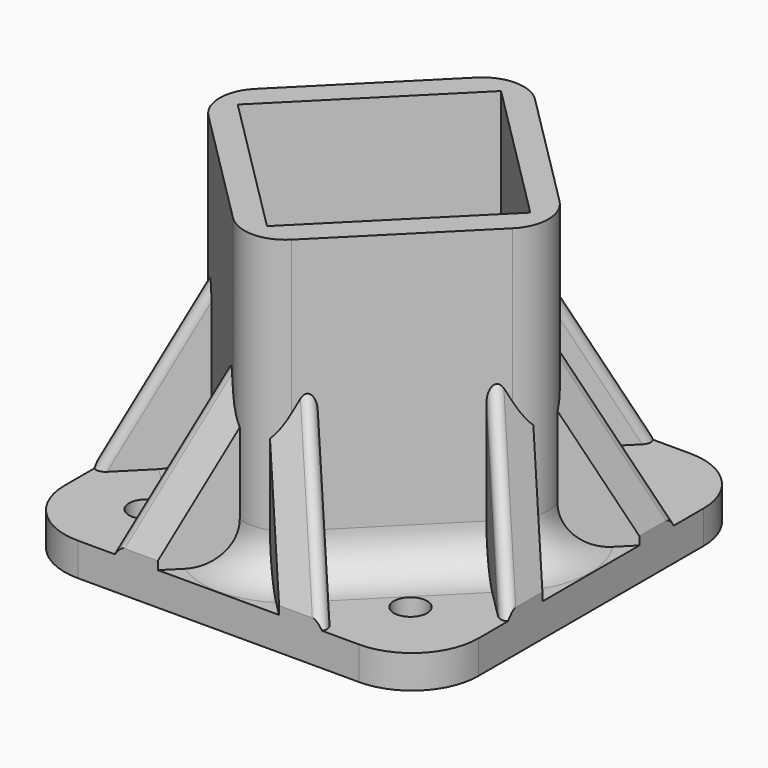
from build123d import *

# Parameters (mm, degrees)
F0_R         = 2
F1_DEPTH     = 4
F0_R_2       = 5
F2_DEPTH     = 40
F3_R         = 8
F4_DEPTH     = 25
F5_T4_DEPTH  = 110.0885065959
F5_T10_DEPTH = 110.0885065959
F5_T16_DEPTH = 110.0885065959
F5_T22_DEPTH = 110.0885065959
F5_T28_DEPTH = 110.0885065959
F5_T34_DEPTH = 110.0885065959
F5_T40_DEPTH = 110.0885065959
F5_T46_DEPTH = 110.0885065959
F5_T52_DEPTH = 110.0885065959
F5_T58_DEPTH = 110.0885065959
F5_T64_DEPTH = 110.0885065959
F5_T70_DEPTH = 110.0885065959
F6_T4_DEPTH  = 110.0885065959
F6_T10_DEPTH = 110.0885065959
F6_T16_DEPTH = 110.0885065959
F6_T22_DEPTH = 110.0885065959
F6_T28_DEPTH = 110.0885065959
F6_T34_DEPTH = 110.0885065959
F6_T40_DEPTH = 110.0885065959
F6_T46_DEPTH = 110.0885065959
F6_T52_DEPTH = 110.0885065959
F6_T58_DEPTH = 110.0885065959
F6_T64_DEPTH = 110.0885065959
F6_T70_DEPTH = 110.0885065959
F7_T4_DEPTH  = 33.9588716378
F7_T10_DEPTH = 33.9588716378
F7_T16_DEPTH = 33.9588716378
F7_T22_DEPTH = 33.9588716378
F7_T28_DEPTH = 33.9588716378
F7_T34_DEPTH = 33.9588716378
F7_T40_DEPTH = 33.9588716378
F7_T46_DEPTH = 33.9588716378
F8_R         = 5
F9_R         = 5


# Not quite as in the source:
# - a fillet or chamfer that OpenCascade refuses, or shapes differently, is made with other operations: its cross-section is extruded or revolved along the edge and cut away or added


with BuildPart() as f1:
    # F0 (on Top) → F1 (new body)
    with BuildSketch(Plane.XY):
        Polygon((16.6170093579, 5.3033008589), (25, 13.686291501), (25, 25), (13.686291501, 25), (5.3033008589, 16.6170093579), align=None)
        with Locations((16, 16)):
            Circle(F0_R, mode=Mode.SUBTRACT)
        Polygon((19.7989898732, -2.1213203436), (25, -7.3223304703), (25, 7.3223304703), (19.7989898732, 2.1213203436), (21.9203102168, 0), align=None)
        Polygon((13.686291501, -25), (25, -25), (25, -13.686291501), (16.6170093579, -5.3033008589), (5.3033008589, -16.6170093579), align=None)
        with Locations((16, -16)):
            Circle(F0_R, mode=Mode.SUBTRACT)
        Polygon((-7.3223304703, -25), (7.3223304703, -25), (2.1213203436, -19.7989898732), (0, -21.9203102168), (-2.1213203436, -19.7989898732), align=None)
        Polygon((-25, -25), (-13.686291501, -25), (-5.3033008589, -16.6170093579), (-16.6170093579, -5.3033008589), (-25, -13.686291501), align=None)
        with Locations((-16, -16)):
            Circle(F0_R, mode=Mode.SUBTRACT)
        Polygon((-25, 7.3223304703), (-25, -7.3223304703), (-19.7989898732, -2.1213203436), (-21.9203102168, 0), (-19.7989898732, 2.1213203436), align=None)
        Polygon((-25, 25), (-25, 13.686291501), (-16.6170093579, 5.3033008589), (-5.3033008589, 16.6170093579), (-13.686291501, 25), align=None)
        with Locations((-16, 16)):
            Circle(F0_R, mode=Mode.SUBTRACT)
        Polygon((-2.1213203436, 19.7989898732), (-7.3223304703, 25), (-13.686291501, 25), (-5.3033008589, 16.6170093579), align=None)
        Polygon((2.1213203436, 19.7989898732), (7.3223304703, 25), (-7.3223304703, 25), (-2.1213203436, 19.7989898732), (0, 21.9203102168), align=None)
        Polygon((5.3033008589, 16.6170093579), (13.686291501, 25), (7.3223304703, 25), (2.1213203436, 19.7989898732), align=None)
        Polygon((19.7989898732, 2.1213203436), (25, 7.3223304703), (25, 13.686291501), (16.6170093579, 5.3033008589), align=None)
        Polygon((16.6170093579, -5.3033008589), (25, -13.686291501), (25, -7.3223304703), (19.7989898732, -2.1213203436), align=None)
        Polygon((7.3223304703, -25), (13.686291501, -25), (5.3033008589, -16.6170093579), (2.1213203436, -19.7989898732), align=None)
        Polygon((-13.686291501, -25), (-7.3223304703, -25), (-2.1213203436, -19.7989898732), (-5.3033008589, -16.6170093579), align=None)
        Polygon((-25, -7.3223304703), (-25, -13.686291501), (-16.6170093579, -5.3033008589), (-19.7989898732, -2.1213203436), align=None)
        Polygon((-25, 13.686291501), (-25, 7.3223304703), (-19.7989898732, 2.1213203436), (-16.6170093579, 5.3033008589), align=None)
    extrude(amount=F1_DEPTH)



with BuildPart() as f1b:
    # F0 (on Top) → F1, piece 2 (new body)
    with BuildSketch(Plane.XY):
        Polygon((0, -17.6776695297), (17.6776695297, 0), (0, 17.6776695297), (-17.6776695297, 0), align=None)
        Circle(F0_R_2, mode=Mode.SUBTRACT)
    extrude(amount=F1_DEPTH)


with BuildPart() as f1_1:
    add(f1.part)

    add(f1b.part)  # F2 merges F1b
    # F0 (on Top) → F2 (join)
    with BuildSketch(Plane.XY):
        Polygon((2.1213203436, -19.7989898732), (5.3033008589, -16.6170093579), (16.6170093579, -5.3033008589), (19.7989898732, -2.1213203436), (21.9203102168, 0), (19.7989898732, 2.1213203436), (16.6170093579, 5.3033008589), (5.3033008589, 16.6170093579), (2.1213203436, 19.7989898732), (0, 21.9203102168), (-2.1213203436, 19.7989898732), (-5.3033008589, 16.6170093579), (-16.6170093579, 5.3033008589), (-19.7989898732, 2.1213203436), (-21.9203102168, 0), (-19.7989898732, -2.1213203436), (-16.6170093579, -5.3033008589), (-5.3033008589, -16.6170093579), (-2.1213203436, -19.7989898732), (0, -21.9203102168), align=None)
        Polygon((0, 17.6776695297), (17.6776695297, 0), (0, -17.6776695297), (-17.6776695297, 0), align=None, mode=Mode.SUBTRACT)
    extrude(amount=F2_DEPTH)

    # F3
    f3_edges = [f1_1.edges().sort_by_distance(p)[0] for p in [
        (-25, 25, 2),
        (-25, -25, 2),
        (25, -25, 2),
        (25, 25, 2),
    ]]
    fillet(f3_edges, radius=F3_R)

    # F0 (on Top) → F4 (join)
    with BuildSketch(Plane.XY):
        Polygon((16.6170093579, -5.3033008589), (25, -13.686291501), (25, -7.3223304703), (19.7989898732, -2.1213203436), align=None)
        Polygon((7.3223304703, -25), (13.686291501, -25), (5.3033008589, -16.6170093579), (2.1213203436, -19.7989898732), align=None)
        Polygon((5.3033008589, 16.6170093579), (13.686291501, 25), (7.3223304703, 25), (2.1213203436, 19.7989898732), align=None)
        Polygon((19.7989898732, 2.1213203436), (25, 7.3223304703), (25, 13.686291501), (16.6170093579, 5.3033008589), align=None)
        Polygon((-13.686291501, -25), (-7.3223304703, -25), (-2.1213203436, -19.7989898732), (-5.3033008589, -16.6170093579), align=None)
        Polygon((-25, -7.3223304703), (-25, -13.686291501), (-16.6170093579, -5.3033008589), (-19.7989898732, -2.1213203436), align=None)
        Polygon((-25, 13.686291501), (-25, 7.3223304703), (-19.7989898732, 2.1213203436), (-16.6170093579, 5.3033008589), align=None)
        Polygon((-2.1213203436, 19.7989898732), (-7.3223304703, 25), (-13.686291501, 25), (-5.3033008589, 16.6170093579), align=None)
    extrude(amount=F4_DEPTH)

    # F5: chamfer of 20 x 8 on 4 edges, made by hand


with BuildPart() as f5_tool2:
    # F5_s3 → F5_t4 (new body)
    with BuildSketch(Plane.YZ.offset(-65.5485642836)):
        Polygon((-17, 25), (-25, 5), (-25, 25), align=None)
    extrude(amount=F5_T4_DEPTH)

    split(bisect_by=Plane(origin=(-10.9601551084, -10.9601551084, 0), x_dir=(0, 0, 1), z_dir=(-0.7071067812, -0.7071067812, 0)), keep=Keep.TOP)

    split(bisect_by=Plane(origin=(10.9601551084, -10.9601551084, 0), x_dir=(0, 0, 1), z_dir=(-0.7071067812, 0.7071067812, 0)), keep=Keep.TOP)


with BuildPart() as f1_2:
    add(f1_1.part)

    # F5_t1: cut F5_tool2
    add(f5_tool2.part, mode=Mode.SUBTRACT)


with BuildPart() as f5_tool8:
    # F5_s9 → F5_t10 (new body)
    with BuildSketch(Plane.YZ.offset(-65.5485642836)):
        Polygon((-17, 25), (-25, 5), (-25, 25), align=None)
    extrude(amount=F5_T10_DEPTH)

    split(bisect_by=Plane(origin=(-10.9601551084, -10.9601551084, 0), x_dir=(0, 0, 1), z_dir=(-0.7071067812, -0.7071067812, 0)), keep=Keep.TOP)

    split(bisect_by=Plane(origin=(10.9601551084, -10.9601551084, 0), x_dir=(0, 0, 1), z_dir=(0.7071067812, -0.7071067812, 0)), keep=Keep.TOP)


with BuildPart() as f1_3:
    add(f1_2.part)

    # F5_t7: cut F5_tool8
    add(f5_tool8.part, mode=Mode.SUBTRACT)


with BuildPart() as f5_tool14:
    # F5_s15 → F5_t16 (new body)
    with BuildSketch(Plane.YZ.offset(-65.5485642836)):
        Polygon((-17, 25), (-25, 5), (-25, 25), align=None)
    extrude(amount=F5_T16_DEPTH)

    split(bisect_by=Plane(origin=(-10.9601551084, -10.9601551084, 0), x_dir=(0, 0, 1), z_dir=(0.7071067812, 0.7071067812, 0)), keep=Keep.TOP)

    split(bisect_by=Plane(origin=(10.9601551084, -10.9601551084, 0), x_dir=(0, 0, 1), z_dir=(0.7071067812, -0.7071067812, 0)), keep=Keep.TOP)


with BuildPart() as f1_4:
    add(f1_3.part)

    # F5_t13: cut F5_tool14
    add(f5_tool14.part, mode=Mode.SUBTRACT)


with BuildPart() as f5_tool20:
    # F5_s21 → F5_t22 (new body)
    with BuildSketch(Plane.YZ.offset(-44.5399423123)):
        Polygon((-17, 25), (-25, 5), (-25, 25), align=None)
    extrude(amount=F5_T22_DEPTH)

    split(bisect_by=Plane(origin=(-10.9601551084, -10.9601551084, 0), x_dir=(0, 0, 1), z_dir=(-0.7071067812, -0.7071067812, 0)), keep=Keep.TOP)

    split(bisect_by=Plane(origin=(10.9601551084, -10.9601551084, 0), x_dir=(0, 0, 1), z_dir=(-0.7071067812, 0.7071067812, 0)), keep=Keep.TOP)


with BuildPart() as f1_5:
    add(f1_4.part)

    # F5_t19: cut F5_tool20
    add(f5_tool20.part, mode=Mode.SUBTRACT)


with BuildPart() as f5_tool26:
    # F5_s27 → F5_t28 (new body)
    with BuildSketch(Plane.YZ.offset(-44.5399423123)):
        Polygon((-17, 25), (-25, 5), (-25, 25), align=None)
    extrude(amount=F5_T28_DEPTH)

    split(bisect_by=Plane(origin=(-10.9601551084, -10.9601551084, 0), x_dir=(0, 0, 1), z_dir=(-0.7071067812, -0.7071067812, 0)), keep=Keep.TOP)

    split(bisect_by=Plane(origin=(10.9601551084, -10.9601551084, 0), x_dir=(0, 0, 1), z_dir=(0.7071067812, -0.7071067812, 0)), keep=Keep.TOP)


with BuildPart() as f1_6:
    add(f1_5.part)

    # F5_t25: cut F5_tool26
    add(f5_tool26.part, mode=Mode.SUBTRACT)


with BuildPart() as f5_tool32:
    # F5_s33 → F5_t34 (new body)
    with BuildSketch(Plane.YZ.offset(-44.5399423123)):
        Polygon((-17, 25), (-25, 5), (-25, 25), align=None)
    extrude(amount=F5_T34_DEPTH)

    split(bisect_by=Plane(origin=(-10.9601551084, -10.9601551084, 0), x_dir=(0, 0, 1), z_dir=(0.7071067812, 0.7071067812, 0)), keep=Keep.TOP)

    split(bisect_by=Plane(origin=(10.9601551084, -10.9601551084, 0), x_dir=(0, 0, 1), z_dir=(0.7071067812, -0.7071067812, 0)), keep=Keep.TOP)


with BuildPart() as f1_7:
    add(f1_6.part)

    # F5_t31: cut F5_tool32
    add(f5_tool32.part, mode=Mode.SUBTRACT)


with BuildPart() as f5_tool38:
    # F5_s39 → F5_t40 (new body)
    with BuildSketch(Plane.XZ.offset(-65.5485642836)):
        Polygon((-17, 25), (-25, 5), (-25, 25), align=None)
    extrude(amount=F5_T40_DEPTH)

    split(bisect_by=Plane(origin=(-10.9601551084, 10.9601551084, 0), x_dir=(0, 0, 1), z_dir=(-0.7071067812, 0.7071067812, 0)), keep=Keep.TOP)

    split(bisect_by=Plane(origin=(-10.9601551084, -10.9601551084, 0), x_dir=(0, 0, 1), z_dir=(0.7071067812, 0.7071067812, 0)), keep=Keep.TOP)


with BuildPart() as f1_8:
    add(f1_7.part)

    # F5_t37: cut F5_tool38
    add(f5_tool38.part, mode=Mode.SUBTRACT)


with BuildPart() as f5_tool44:
    # F5_s45 → F5_t46 (new body)
    with BuildSketch(Plane.XZ.offset(-65.5485642836)):
        Polygon((-17, 25), (-25, 5), (-25, 25), align=None)
    extrude(amount=F5_T46_DEPTH)

    split(bisect_by=Plane(origin=(-10.9601551084, 10.9601551084, 0), x_dir=(0, 0, 1), z_dir=(-0.7071067812, 0.7071067812, 0)), keep=Keep.TOP)

    split(bisect_by=Plane(origin=(-10.9601551084, -10.9601551084, 0), x_dir=(0, 0, 1), z_dir=(-0.7071067812, -0.7071067812, 0)), keep=Keep.TOP)


with BuildPart() as f1_9:
    add(f1_8.part)

    # F5_t43: cut F5_tool44
    add(f5_tool44.part, mode=Mode.SUBTRACT)


with BuildPart() as f5_tool50:
    # F5_s51 → F5_t52 (new body)
    with BuildSketch(Plane.XZ.offset(-65.5485642836)):
        Polygon((-17, 25), (-25, 5), (-25, 25), align=None)
    extrude(amount=F5_T52_DEPTH)

    split(bisect_by=Plane(origin=(-10.9601551084, 10.9601551084, 0), x_dir=(0, 0, 1), z_dir=(0.7071067812, -0.7071067812, 0)), keep=Keep.TOP)

    split(bisect_by=Plane(origin=(-10.9601551084, -10.9601551084, 0), x_dir=(0, 0, 1), z_dir=(-0.7071067812, -0.7071067812, 0)), keep=Keep.TOP)


with BuildPart() as f1_10:
    add(f1_9.part)

    # F5_t49: cut F5_tool50
    add(f5_tool50.part, mode=Mode.SUBTRACT)


with BuildPart() as f5_tool56:
    # F5_s57 → F5_t58 (new body)
    with BuildSketch(Plane.XZ.offset(-44.5399423123)):
        Polygon((-17, 25), (-25, 5), (-25, 25), align=None)
    extrude(amount=F5_T58_DEPTH)

    split(bisect_by=Plane(origin=(-10.9601551084, 10.9601551084, 0), x_dir=(0, 0, 1), z_dir=(-0.7071067812, 0.7071067812, 0)), keep=Keep.TOP)

    split(bisect_by=Plane(origin=(-10.9601551084, -10.9601551084, 0), x_dir=(0, 0, 1), z_dir=(0.7071067812, 0.7071067812, 0)), keep=Keep.TOP)


with BuildPart() as f1_11:
    add(f1_10.part)

    # F5_t55: cut F5_tool56
    add(f5_tool56.part, mode=Mode.SUBTRACT)


with BuildPart() as f5_tool62:
    # F5_s63 → F5_t64 (new body)
    with BuildSketch(Plane.XZ.offset(-44.5399423123)):
        Polygon((-17, 25), (-25, 5), (-25, 25), align=None)
    extrude(amount=F5_T64_DEPTH)

    split(bisect_by=Plane(origin=(-10.9601551084, 10.9601551084, 0), x_dir=(0, 0, 1), z_dir=(-0.7071067812, 0.7071067812, 0)), keep=Keep.TOP)

    split(bisect_by=Plane(origin=(-10.9601551084, -10.9601551084, 0), x_dir=(0, 0, 1), z_dir=(-0.7071067812, -0.7071067812, 0)), keep=Keep.TOP)


with BuildPart() as f1_12:
    add(f1_11.part)

    # F5_t61: cut F5_tool62
    add(f5_tool62.part, mode=Mode.SUBTRACT)


with BuildPart() as f5_tool68:
    # F5_s69 → F5_t70 (new body)
    with BuildSketch(Plane.XZ.offset(-44.5399423123)):
        Polygon((-17, 25), (-25, 5), (-25, 25), align=None)
    extrude(amount=F5_T70_DEPTH)

    split(bisect_by=Plane(origin=(-10.9601551084, 10.9601551084, 0), x_dir=(0, 0, 1), z_dir=(0.7071067812, -0.7071067812, 0)), keep=Keep.TOP)

    split(bisect_by=Plane(origin=(-10.9601551084, -10.9601551084, 0), x_dir=(0, 0, 1), z_dir=(-0.7071067812, -0.7071067812, 0)), keep=Keep.TOP)


with BuildPart() as f1_13:
    add(f1_12.part)

    # F5_t67: cut F5_tool68
    add(f5_tool68.part, mode=Mode.SUBTRACT)

    # F6: chamfer of 8 x 20 on 4 edges, made by hand


with BuildPart() as f6_tool2:
    # F6_s3 → F6_t4 (new body)
    with BuildSketch(Plane.XZ.offset(65.5485642836)):
        Polygon((17, 25), (25, 5), (25, 25), align=None)
    extrude(amount=-F6_T4_DEPTH)

    split(bisect_by=Plane(origin=(10.9601551084, -10.9601551084, 0), x_dir=(0, 0, 1), z_dir=(0.7071067812, -0.7071067812, 0)), keep=Keep.TOP)

    split(bisect_by=Plane(origin=(10.9601551084, 10.9601551084, 0), x_dir=(0, 0, 1), z_dir=(-0.7071067812, -0.7071067812, 0)), keep=Keep.TOP)


with BuildPart() as f1_14:
    add(f1_13.part)

    # F6_t1: cut F6_tool2
    add(f6_tool2.part, mode=Mode.SUBTRACT)


with BuildPart() as f6_tool8:
    # F6_s9 → F6_t10 (new body)
    with BuildSketch(Plane.XZ.offset(65.5485642836)):
        Polygon((17, 25), (25, 5), (25, 25), align=None)
    extrude(amount=-F6_T10_DEPTH)

    split(bisect_by=Plane(origin=(10.9601551084, -10.9601551084, 0), x_dir=(0, 0, 1), z_dir=(0.7071067812, -0.7071067812, 0)), keep=Keep.TOP)

    split(bisect_by=Plane(origin=(10.9601551084, 10.9601551084, 0), x_dir=(0, 0, 1), z_dir=(0.7071067812, 0.7071067812, 0)), keep=Keep.TOP)


with BuildPart() as f1_15:
    add(f1_14.part)

    # F6_t7: cut F6_tool8
    add(f6_tool8.part, mode=Mode.SUBTRACT)


with BuildPart() as f6_tool14:
    # F6_s15 → F6_t16 (new body)
    with BuildSketch(Plane.XZ.offset(65.5485642836)):
        Polygon((17, 25), (25, 5), (25, 25), align=None)
    extrude(amount=-F6_T16_DEPTH)

    split(bisect_by=Plane(origin=(10.9601551084, -10.9601551084, 0), x_dir=(0, 0, 1), z_dir=(-0.7071067812, 0.7071067812, 0)), keep=Keep.TOP)

    split(bisect_by=Plane(origin=(10.9601551084, 10.9601551084, 0), x_dir=(0, 0, 1), z_dir=(0.7071067812, 0.7071067812, 0)), keep=Keep.TOP)


with BuildPart() as f1_16:
    add(f1_15.part)

    # F6_t13: cut F6_tool14
    add(f6_tool14.part, mode=Mode.SUBTRACT)


with BuildPart() as f6_tool20:
    # F6_s21 → F6_t22 (new body)
    with BuildSketch(Plane.XZ.offset(44.5399423123)):
        Polygon((17, 25), (25, 5), (25, 25), align=None)
    extrude(amount=-F6_T22_DEPTH)

    split(bisect_by=Plane(origin=(10.9601551084, -10.9601551084, 0), x_dir=(0, 0, 1), z_dir=(0.7071067812, -0.7071067812, 0)), keep=Keep.TOP)

    split(bisect_by=Plane(origin=(10.9601551084, 10.9601551084, 0), x_dir=(0, 0, 1), z_dir=(-0.7071067812, -0.7071067812, 0)), keep=Keep.TOP)


with BuildPart() as f1_17:
    add(f1_16.part)

    # F6_t19: cut F6_tool20
    add(f6_tool20.part, mode=Mode.SUBTRACT)


with BuildPart() as f6_tool26:
    # F6_s27 → F6_t28 (new body)
    with BuildSketch(Plane.XZ.offset(44.5399423123)):
        Polygon((17, 25), (25, 5), (25, 25), align=None)
    extrude(amount=-F6_T28_DEPTH)

    split(bisect_by=Plane(origin=(10.9601551084, -10.9601551084, 0), x_dir=(0, 0, 1), z_dir=(0.7071067812, -0.7071067812, 0)), keep=Keep.TOP)

    split(bisect_by=Plane(origin=(10.9601551084, 10.9601551084, 0), x_dir=(0, 0, 1), z_dir=(0.7071067812, 0.7071067812, 0)), keep=Keep.TOP)


with BuildPart() as f1_18:
    add(f1_17.part)

    # F6_t25: cut F6_tool26
    add(f6_tool26.part, mode=Mode.SUBTRACT)


with BuildPart() as f6_tool32:
    # F6_s33 → F6_t34 (new body)
    with BuildSketch(Plane.XZ.offset(44.5399423123)):
        Polygon((17, 25), (25, 5), (25, 25), align=None)
    extrude(amount=-F6_T34_DEPTH)

    split(bisect_by=Plane(origin=(10.9601551084, -10.9601551084, 0), x_dir=(0, 0, 1), z_dir=(-0.7071067812, 0.7071067812, 0)), keep=Keep.TOP)

    split(bisect_by=Plane(origin=(10.9601551084, 10.9601551084, 0), x_dir=(0, 0, 1), z_dir=(0.7071067812, 0.7071067812, 0)), keep=Keep.TOP)


with BuildPart() as f1_19:
    add(f1_18.part)

    # F6_t31: cut F6_tool32
    add(f6_tool32.part, mode=Mode.SUBTRACT)


with BuildPart() as f6_tool38:
    # F6_s39 → F6_t40 (new body)
    with BuildSketch(Plane.YZ.offset(65.5485642836)):
        Polygon((17, 25), (25, 5), (25, 25), align=None)
    extrude(amount=-F6_T40_DEPTH)

    split(bisect_by=Plane(origin=(10.9601551084, 10.9601551084, 0), x_dir=(0, 0, 1), z_dir=(0.7071067812, 0.7071067812, 0)), keep=Keep.TOP)

    split(bisect_by=Plane(origin=(-10.9601551084, 10.9601551084, 0), x_dir=(0, 0, 1), z_dir=(0.7071067812, -0.7071067812, 0)), keep=Keep.TOP)


with BuildPart() as f1_20:
    add(f1_19.part)

    # F6_t37: cut F6_tool38
    add(f6_tool38.part, mode=Mode.SUBTRACT)


with BuildPart() as f6_tool44:
    # F6_s45 → F6_t46 (new body)
    with BuildSketch(Plane.YZ.offset(65.5485642836)):
        Polygon((17, 25), (25, 5), (25, 25), align=None)
    extrude(amount=-F6_T46_DEPTH)

    split(bisect_by=Plane(origin=(10.9601551084, 10.9601551084, 0), x_dir=(0, 0, 1), z_dir=(0.7071067812, 0.7071067812, 0)), keep=Keep.TOP)

    split(bisect_by=Plane(origin=(-10.9601551084, 10.9601551084, 0), x_dir=(0, 0, 1), z_dir=(-0.7071067812, 0.7071067812, 0)), keep=Keep.TOP)


with BuildPart() as f1_21:
    add(f1_20.part)

    # F6_t43: cut F6_tool44
    add(f6_tool44.part, mode=Mode.SUBTRACT)


with BuildPart() as f6_tool50:
    # F6_s51 → F6_t52 (new body)
    with BuildSketch(Plane.YZ.offset(65.5485642836)):
        Polygon((17, 25), (25, 5), (25, 25), align=None)
    extrude(amount=-F6_T52_DEPTH)

    split(bisect_by=Plane(origin=(10.9601551084, 10.9601551084, 0), x_dir=(0, 0, 1), z_dir=(-0.7071067812, -0.7071067812, 0)), keep=Keep.TOP)

    split(bisect_by=Plane(origin=(-10.9601551084, 10.9601551084, 0), x_dir=(0, 0, 1), z_dir=(-0.7071067812, 0.7071067812, 0)), keep=Keep.TOP)


with BuildPart() as f1_22:
    add(f1_21.part)

    # F6_t49: cut F6_tool50
    add(f6_tool50.part, mode=Mode.SUBTRACT)


with BuildPart() as f6_tool56:
    # F6_s57 → F6_t58 (new body)
    with BuildSketch(Plane.YZ.offset(44.5399423123)):
        Polygon((17, 25), (25, 5), (25, 25), align=None)
    extrude(amount=-F6_T58_DEPTH)

    split(bisect_by=Plane(origin=(10.9601551084, 10.9601551084, 0), x_dir=(0, 0, 1), z_dir=(0.7071067812, 0.7071067812, 0)), keep=Keep.TOP)

    split(bisect_by=Plane(origin=(-10.9601551084, 10.9601551084, 0), x_dir=(0, 0, 1), z_dir=(0.7071067812, -0.7071067812, 0)), keep=Keep.TOP)


with BuildPart() as f1_23:
    add(f1_22.part)

    # F6_t55: cut F6_tool56
    add(f6_tool56.part, mode=Mode.SUBTRACT)


with BuildPart() as f6_tool62:
    # F6_s63 → F6_t64 (new body)
    with BuildSketch(Plane.YZ.offset(44.5399423123)):
        Polygon((17, 25), (25, 5), (25, 25), align=None)
    extrude(amount=-F6_T64_DEPTH)

    split(bisect_by=Plane(origin=(10.9601551084, 10.9601551084, 0), x_dir=(0, 0, 1), z_dir=(0.7071067812, 0.7071067812, 0)), keep=Keep.TOP)

    split(bisect_by=Plane(origin=(-10.9601551084, 10.9601551084, 0), x_dir=(0, 0, 1), z_dir=(-0.7071067812, 0.7071067812, 0)), keep=Keep.TOP)


with BuildPart() as f1_24:
    add(f1_23.part)

    # F6_t61: cut F6_tool62
    add(f6_tool62.part, mode=Mode.SUBTRACT)


with BuildPart() as f6_tool68:
    # F6_s69 → F6_t70 (new body)
    with BuildSketch(Plane.YZ.offset(44.5399423123)):
        Polygon((17, 25), (25, 5), (25, 25), align=None)
    extrude(amount=-F6_T70_DEPTH)

    split(bisect_by=Plane(origin=(10.9601551084, 10.9601551084, 0), x_dir=(0, 0, 1), z_dir=(-0.7071067812, -0.7071067812, 0)), keep=Keep.TOP)

    split(bisect_by=Plane(origin=(-10.9601551084, 10.9601551084, 0), x_dir=(0, 0, 1), z_dir=(-0.7071067812, 0.7071067812, 0)), keep=Keep.TOP)


with BuildPart() as f1_25:
    add(f1_24.part)

    # F6_t67: cut F6_tool68
    add(f6_tool68.part, mode=Mode.SUBTRACT)

    # F7: fillet of radius 1 on 8 edges, made by hand


with BuildPart() as f7_tool2:
    # F7_s3 → F7_t4 (new body)
    with BuildSketch(Plane(origin=(-6.7373848341, 6.7373848341, 16.8434620852), x_dir=(0.7071067812, 0.7071067812, 0), z_dir=(0.3481553119, -0.3481553119, -0.8703882798))):
        with BuildLine():
            ThreePointArc((-9.6565321643, 24.8297701453), (-8.5855920876, 24.9855633652), (-8, 24.0754721159))
            Line((-8, 24.0754721159), (-8, 26.2715963262))
            Line((-8, 26.2715963262), (-9.6565321643, 24.8297701453))
        make_face()
    extrude(amount=F7_T4_DEPTH)

    split(bisect_by=Plane(origin=(10.9601551084, -10.9601551084, 0), x_dir=(0, 0, 1), z_dir=(0.7071067812, -0.7071067812, 0)), keep=Keep.TOP)

    split(bisect_by=Plane.XY.offset(4), keep=Keep.TOP)


with BuildPart() as f1_26:
    add(f1_25.part)

    # F7_t1: cut F7_tool2
    add(f7_tool2.part, mode=Mode.SUBTRACT)


with BuildPart() as f7_tool8:
    # F7_s9 → F7_t10 (new body)
    with BuildSketch(Plane(origin=(5.0855767131, -5.0855767131, -12.7139417828), x_dir=(-0.7071067812, -0.7071067812, 0), z_dir=(-0.3481553119, 0.3481553119, 0.8703882798))):
        with BuildLine():
            ThreePointArc((-8, 24.0754721159), (-8.5855920876, 24.9855633652), (-9.6565321643, 24.8297701453))
            Line((-9.6565321643, 24.8297701453), (-8, 26.2715963262))
            Line((-8, 26.2715963262), (-8, 24.0754721159))
        make_face()
    extrude(amount=F7_T10_DEPTH)

    split(bisect_by=Plane(origin=(10.9601551084, -10.9601551084, 0), x_dir=(0, 0, 1), z_dir=(0.7071067812, -0.7071067812, 0)), keep=Keep.TOP)

    split(bisect_by=Plane.XY.offset(4), keep=Keep.TOP)


with BuildPart() as f1_27:
    add(f1_26.part)

    # F7_t7: cut F7_tool8
    add(f7_tool8.part, mode=Mode.SUBTRACT)


with BuildPart() as f7_tool14:
    # F7_s15 → F7_t16 (new body)
    with BuildSketch(Plane(origin=(-6.7373848341, -6.7373848341, 16.8434620852), x_dir=(-0.7071067812, 0.7071067812, 0), z_dir=(0.3481553119, 0.3481553119, -0.8703882798))):
        with BuildLine():
            ThreePointArc((-9.6565321643, 24.8297701453), (-8.5855920876, 24.9855633652), (-8, 24.0754721159))
            Line((-8, 24.0754721159), (-8, 26.2715963262))
            Line((-8, 26.2715963262), (-9.6565321643, 24.8297701453))
        make_face()
    extrude(amount=F7_T16_DEPTH)

    split(bisect_by=Plane.XY.offset(4), keep=Keep.TOP)

    split(bisect_by=Plane(origin=(10.9601551084, 10.9601551084, 0), x_dir=(0, 0, 1), z_dir=(0.7071067812, 0.7071067812, 0)), keep=Keep.TOP)


with BuildPart() as f1_28:
    add(f1_27.part)

    # F7_t13: cut F7_tool14
    add(f7_tool14.part, mode=Mode.SUBTRACT)


with BuildPart() as f7_tool20:
    # F7_s21 → F7_t22 (new body)
    with BuildSketch(Plane(origin=(5.0855767131, 5.0855767131, -12.7139417828), x_dir=(0.7071067812, -0.7071067812, 0), z_dir=(-0.3481553119, -0.3481553119, 0.8703882798))):
        with BuildLine():
            ThreePointArc((-8, 24.0754721159), (-8.5855920876, 24.9855633652), (-9.6565321643, 24.8297701453))
            Line((-9.6565321643, 24.8297701453), (-8, 26.2715963262))
            Line((-8, 26.2715963262), (-8, 24.0754721159))
        make_face()
    extrude(amount=F7_T22_DEPTH)

    split(bisect_by=Plane.XY.offset(4), keep=Keep.TOP)

    split(bisect_by=Plane(origin=(10.9601551084, 10.9601551084, 0), x_dir=(0, 0, 1), z_dir=(0.7071067812, 0.7071067812, 0)), keep=Keep.TOP)


with BuildPart() as f1_29:
    add(f1_28.part)

    # F7_t19: cut F7_tool20
    add(f7_tool20.part, mode=Mode.SUBTRACT)


with BuildPart() as f7_tool26:
    # F7_s27 → F7_t28 (new body)
    with BuildSketch(Plane(origin=(6.7373848341, -6.7373848341, 16.8434620852), x_dir=(-0.7071067812, -0.7071067812, 0), z_dir=(-0.3481553119, 0.3481553119, -0.8703882798))):
        with BuildLine():
            ThreePointArc((-9.6565321643, 24.8297701453), (-8.5855920876, 24.9855633652), (-8, 24.0754721159))
            Line((-8, 24.0754721159), (-8, 26.2715963262))
            Line((-8, 26.2715963262), (-9.6565321643, 24.8297701453))
        make_face()
    extrude(amount=F7_T28_DEPTH)

    split(bisect_by=Plane.XY.offset(4), keep=Keep.TOP)

    split(bisect_by=Plane(origin=(-10.9601551084, 10.9601551084, 0), x_dir=(0, 0, 1), z_dir=(-0.7071067812, 0.7071067812, 0)), keep=Keep.TOP)


with BuildPart() as f1_30:
    add(f1_29.part)

    # F7_t25: cut F7_tool26
    add(f7_tool26.part, mode=Mode.SUBTRACT)


with BuildPart() as f7_tool32:
    # F7_s33 → F7_t34 (new body)
    with BuildSketch(Plane(origin=(-5.0855767131, 5.0855767131, -12.7139417828), x_dir=(0.7071067812, 0.7071067812, 0), z_dir=(0.3481553119, -0.3481553119, 0.8703882798))):
        with BuildLine():
            ThreePointArc((-8, 24.0754721159), (-8.5855920876, 24.9855633652), (-9.6565321643, 24.8297701453))
            Line((-9.6565321643, 24.8297701453), (-8, 26.2715963262))
            Line((-8, 26.2715963262), (-8, 24.0754721159))
        make_face()
    extrude(amount=F7_T34_DEPTH)

    split(bisect_by=Plane.XY.offset(4), keep=Keep.TOP)

    split(bisect_by=Plane(origin=(-10.9601551084, 10.9601551084, 0), x_dir=(0, 0, 1), z_dir=(-0.7071067812, 0.7071067812, 0)), keep=Keep.TOP)


with BuildPart() as f1_31:
    add(f1_30.part)

    # F7_t31: cut F7_tool32
    add(f7_tool32.part, mode=Mode.SUBTRACT)


with BuildPart() as f7_tool38:
    # F7_s39 → F7_t40 (new body)
    with BuildSketch(Plane(origin=(6.7373848341, 6.7373848341, 16.8434620852), x_dir=(0.7071067812, -0.7071067812, 0), z_dir=(-0.3481553119, -0.3481553119, -0.8703882798))):
        with BuildLine():
            ThreePointArc((-9.6565321643, 24.8297701453), (-8.5855920876, 24.9855633652), (-8, 24.0754721159))
            Line((-8, 24.0754721159), (-8, 26.2715963262))
            Line((-8, 26.2715963262), (-9.6565321643, 24.8297701453))
        make_face()
    extrude(amount=F7_T40_DEPTH)

    split(bisect_by=Plane.XY.offset(4), keep=Keep.TOP)

    split(bisect_by=Plane(origin=(-10.9601551084, -10.9601551084, 0), x_dir=(0, 0, 1), z_dir=(-0.7071067812, -0.7071067812, 0)), keep=Keep.TOP)


with BuildPart() as f1_32:
    add(f1_31.part)

    # F7_t37: cut F7_tool38
    add(f7_tool38.part, mode=Mode.SUBTRACT)


with BuildPart() as f7_tool44:
    # F7_s45 → F7_t46 (new body)
    with BuildSketch(Plane(origin=(-5.0855767131, -5.0855767131, -12.7139417828), x_dir=(-0.7071067812, 0.7071067812, 0), z_dir=(0.3481553119, 0.3481553119, 0.8703882798))):
        with BuildLine():
            ThreePointArc((-8, 24.0754721159), (-8.5855920876, 24.9855633652), (-9.6565321643, 24.8297701453))
            Line((-9.6565321643, 24.8297701453), (-8, 26.2715963262))
            Line((-8, 26.2715963262), (-8, 24.0754721159))
        make_face()
    extrude(amount=F7_T46_DEPTH)

    split(bisect_by=Plane.XY.offset(4), keep=Keep.TOP)

    split(bisect_by=Plane(origin=(-10.9601551084, -10.9601551084, 0), x_dir=(0, 0, 1), z_dir=(-0.7071067812, -0.7071067812, 0)), keep=Keep.TOP)


with BuildPart() as f1_33:
    add(f1_32.part)

    # F7_t43: cut F7_tool44
    add(f7_tool44.part, mode=Mode.SUBTRACT)

    # F8
    f8_edges = [f1_33.edges().sort_by_distance(p)[0] for p in [
        (0, -21.92031, 22),
        (21.92031, 0, 22),
        (0, 21.92031, 22),
        (-21.92031, 0, 22),
    ]]
    fillet(f8_edges, radius=F8_R)

    # F9
    f9_edges = [f1_33.edges().sort_by_distance(p)[0] for p in [
        (10.960155, 10.960155, 4),
        (-10.960155, 10.960155, 4),
        (-19.849242, 0, 4),
        (0, 19.849242, 4),
        (-10.960155, -10.960155, 4),
        (0, -19.849242, 4),
        (10.960155, -10.960155, 4),
        (19.849242, 0, 4),
    ]]
    fillet(f9_edges, radius=F9_R)


solid = f1_33.part
